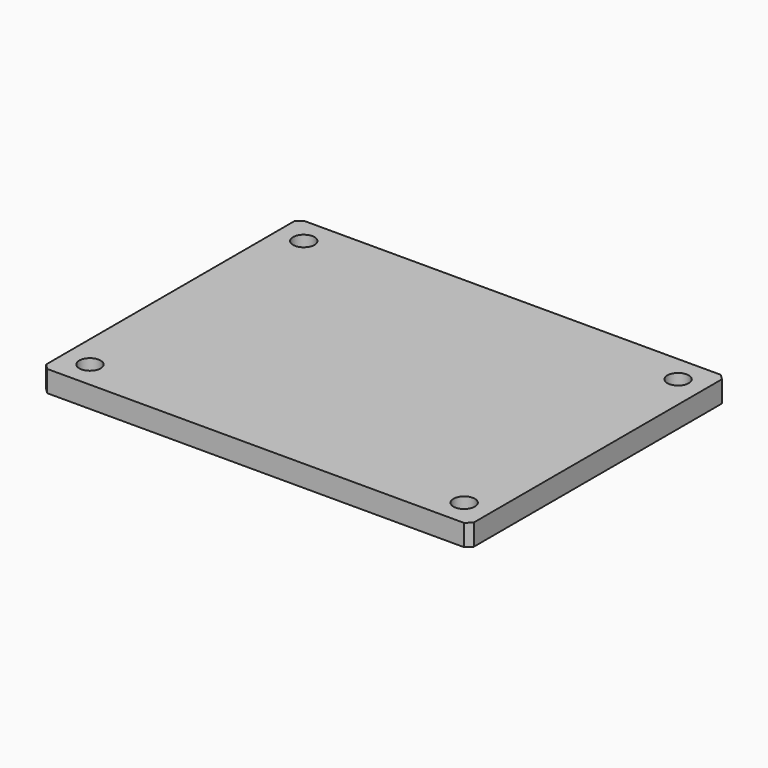
from build123d import *

# Parameters (mm, degrees)
F0_W     = 4000
F0_H     = 3000
F1_DEPTH = 100
F2_SIZE  = 50
F4_D     = 200


with BuildPart() as f1:
    # F0 (on Top) → F1 (new body, symmetric)
    with BuildSketch(Plane.XY):
        Rectangle(F0_W, F0_H)
    extrude(amount=F1_DEPTH, both=True)

    # F2
    f2_edges = [f1.edges().sort_by_distance(p)[0] for p in [
        (-2000, -1500, 0),
        (2000, 1500, 0),
        (2000, -1500, 0),
        (-2000, 1500, 0),
    ]]
    chamfer(f2_edges, length=F2_SIZE)

    # F4 (through all)
    with Locations(Plane.XY.offset(100)):
        with Locations((-1750, 1250), (1750, 1250), (-1750, -1250), (1750, -1250)):
            Hole(F4_D / 2)


solid = f1.part
